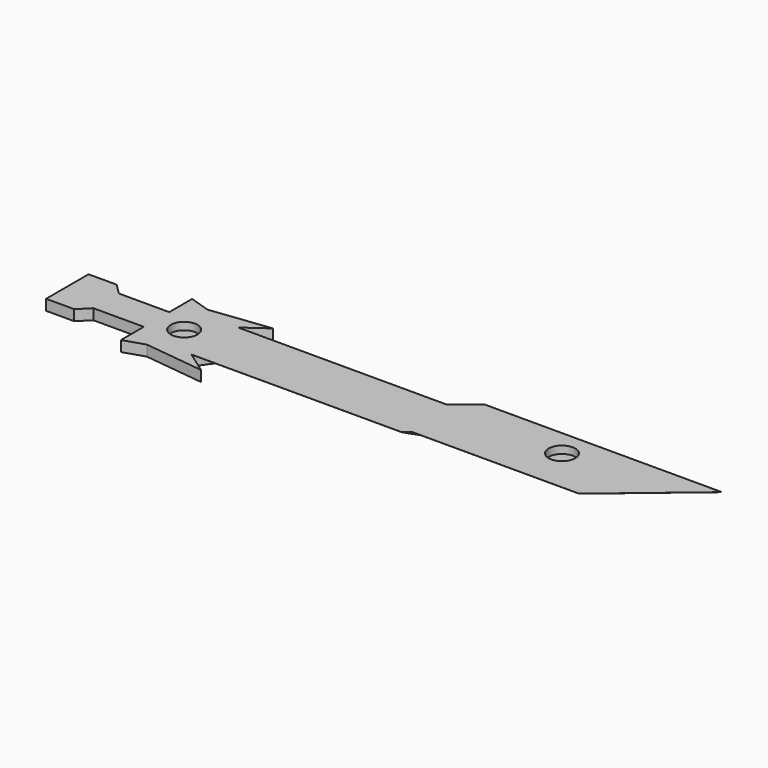
from build123d import *

# Parameters (mm, degrees)
F1_DEPTH = 2
F2_DEPTH = 1.5
F3_SIZE2 = 5
F3_SIZE  = 1.49
F4_SIZE2 = 5
F4_SIZE  = 1.49
F5_SIZE2 = 5
F5_SIZE  = 1.49
F6_SIZE  = 1.99999
F7_R     = 2.5
F8_DEPTH = 1.4


# Not quite as in the source:
# - a fillet or chamfer is up to 0.001 mm smaller than in the source, because OpenCascade refuses the exact size


with BuildPart() as f1:
    # F0 (on Top) → F1 (new body)
    with BuildSketch(Plane.XY):
        Polygon((0, 5), (0, 0), (0, -5), (7.3, -5), (7.3, -3), (16.8, -3), (16.8, -8.3876634017), (20.6713799321, -7.1317504184), (31.9639886349, -8.4706461057), (27.770944377, -5.5), (31.6675294298, 0), (27.770944377, 5.5), (31.9639886349, 8.4706461057), (20.6713799321, 7.1317504184), (16.8, 8.3876634017), (16.8, 3), (7.3, 3), (7.3, 5), align=None)
    extrude(amount=-F1_DEPTH)

    # F0 (on Top) → F2 (join)
    with BuildSketch(Plane.XY):
        Polygon((0, 5), (0, 0), (0, -5), (7.3, -5), (7.3, -3), (16.8, -3), (16.8, -8.3876634017), (20.6713799321, -7.1317504184), (31.9639886349, -8.4706461057), (27.770944377, -5.5), (31.6675294298, 0), (27.770944377, 5.5), (31.9639886349, 8.4706461057), (20.6713799321, 7.1317504184), (16.8, 8.3876634017), (16.8, 3), (7.3, 3), (7.3, 5), align=None)
        Polygon((67.1471691582, 5.5), (27.770944377, 5.5), (31.6675294298, 0), (27.770944377, -5.5), (67.4096829149, -5.5), (68.6014365075, -4.5), (100, -4.5), (116.0886735, 9), (71.3183067322, 9), align=None)
    extrude(amount=-F2_DEPTH)

    # F3
    f3_edges = [f1.edges().sort_by_distance(p)[0] for p in [
        (84.300718, -4.5, -1.5),
    ]]
    f3_side = f1.faces().sort_by_distance((84.300718, -4.5, -0.75))[0]
    chamfer(f3_edges, length=F3_SIZE, length2=F3_SIZE2, reference=f3_side)

    # F4
    f4_edges = [f1.edges().sort_by_distance(p)[0] for p in [
        (47.590314, -5.5, -1.5),
    ]]
    f4_side = f1.faces().sort_by_distance((47.590314, -5.5, -0.75))[0]
    chamfer(f4_edges, length=F4_SIZE, length2=F4_SIZE2, reference=f4_side)

    # F5
    f5_edges = [f1.edges().sort_by_distance(p)[0] for p in [
        (111.023721, 4.75, -1.5),
    ]]
    f5_side = f1.faces().sort_by_distance((109.409925, 3.395865, -0.692895))[0]
    chamfer(f5_edges, length=F5_SIZE, length2=F5_SIZE2, reference=f5_side)

    # F6 (size 2 in the source; OpenCascade refuses exactly that, so slightly less here)
    f6_edges = [f1.edges().sort_by_distance(p)[0] for p in [
        (7.3, 5, -1),
        (7.3, -5, -1),
    ]]
    chamfer(f6_edges, length=F6_SIZE)

    # F7 (on Top) → F8 (cut)
    with BuildSketch(Plane.XY):
        with Locations((22, 0)):
            Circle(F7_R)
        with Locations((90, 3.9548357017)):
            Circle(F7_R)
    extrude(amount=-F8_DEPTH, mode=Mode.SUBTRACT)


solid = f1.part
